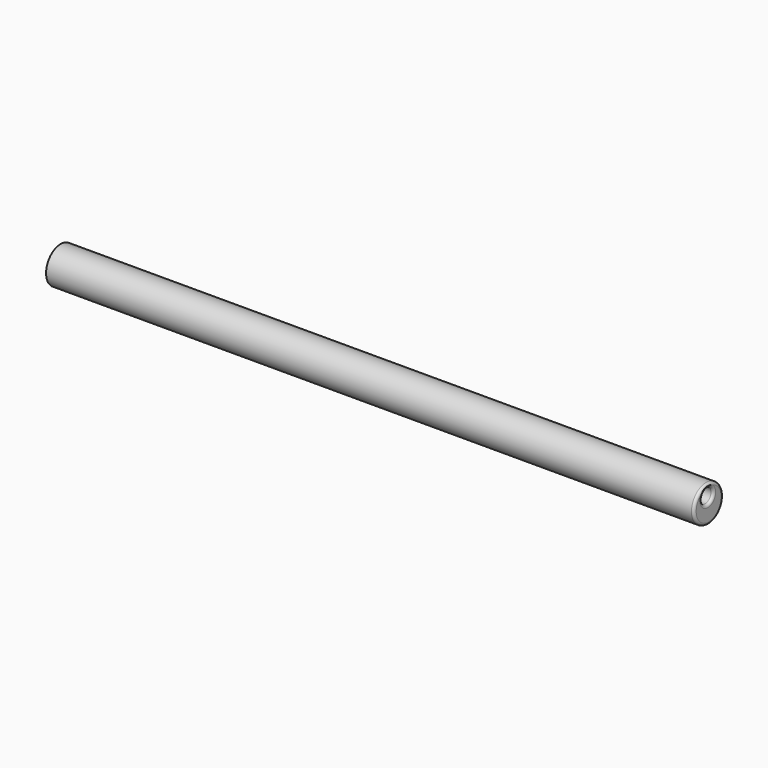
from build123d import *

# Parameters (mm, degrees)
F0_R     = 21.4571011733
F0_R_2   = 8.5102706454
F1_DEPTH = 762


# Not quite as in the source:
# - a fillet or chamfer that OpenCascade refuses, or shapes differently, is made with other operations: its cross-section is extruded or revolved along the edge and cut away or added


with BuildPart() as f1:
    # F0 (on Right) → F1 (new body)
    with BuildSketch(Plane.YZ):
        with Locations((-28.4389311976, 21.4029382453)):
            Circle(F0_R)
        with Locations((-29.8031512648, 29.8031531274)):
            Circle(F0_R_2, mode=Mode.SUBTRACT)
    extrude(amount=F1_DEPTH)

    # F2: fillet of radius 3.0660512242 on 4 edges, made by hand


with BuildPart() as f2_tool1:
    # F2_s2 → F2_t3 (revolve)
    with BuildSketch(Plane.XY.offset(21.4029382453)):
        with BuildLine():
            ThreePointArc((758.9339487758, -6.9818300243), (761.1019743879, -7.8798556364), (762, -10.0478812485))
            Line((762, -10.0478812485), (762, -6.9818300243))
            Line((762, -6.9818300243), (758.9339487758, -6.9818300243))
        make_face()
    revolve(axis=Axis((762, -28.4389311976, 21.4029382453), (1, 0, 0)))


with BuildPart() as f2_tool4:
    # F2_s5 → F2_t6 (revolve)
    with BuildSketch(Plane.XY.offset(29.8031531274)):
        with BuildLine():
            ThreePointArc((758.9339487758, -21.2928806194), (761.1019743879, -20.3948550073), (762, -18.2268293951))
            Line((762, -18.2268293951), (762, -21.2928806194))
            Line((762, -21.2928806194), (758.9339487758, -21.2928806194))
        make_face()
    revolve(axis=Axis((762, -29.8031512648, 29.8031531274), (1, 0, 0)))


with BuildPart() as f2_tool7:
    # F2_s8 → F2_t9 (revolve)
    with BuildSketch(Plane.XY.offset(29.8031531274)):
        with BuildLine():
            ThreePointArc((3.0660512242, -21.2928806194), (0.8980256121, -20.3948550073), (0, -18.2268293951))
            Line((0, -18.2268293951), (0, -21.2928806194))
            Line((0, -21.2928806194), (3.0660512242, -21.2928806194))
        make_face()
    revolve(axis=Axis((0, -29.8031512648, 29.8031531274), (1, 0, 0)))


with BuildPart() as f1_1:
    add(f1.part)

    # F2_t10: cut F2_tool1, F2_tool4, F2_tool7
    add([f2_tool1.part, f2_tool4.part, f2_tool7.part], mode=Mode.SUBTRACT)


solid = f1_1.part
